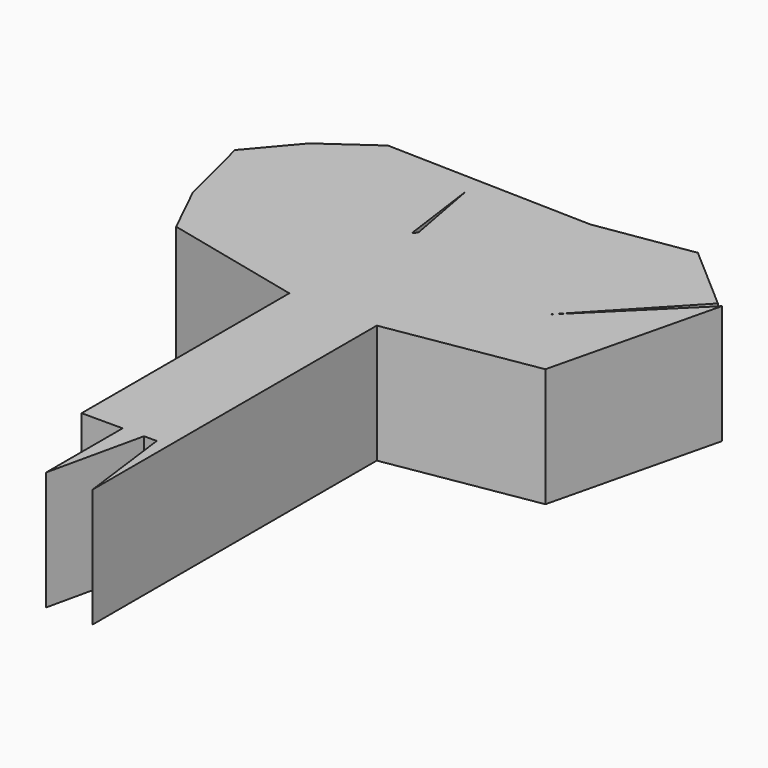
from build123d import *

# Parameters (mm, degrees)
F1_DEPTH = 25.4


with BuildPart() as f1:
    # F0 (on Top) → F1 (new body)
    with BuildSketch(Plane.XY):
        Polygon((-9.9282488227, 16.6444163769), (-9.9282488227, -38.8369709253), (-6.8141991987, -38.8369709253), (-4.3801111169, -38.8369709253), (-1.1680317111, -38.8369709253), (3.4067514008, -38.8369709253), (6.1321551912, -38.8369709253), (8.7602203712, -38.8369709253), (8.7602203712, 16.6444163769), (0, 16.6444163769), (-3.5040895455, 16.6444163769), (-6.8141991987, 16.6444163769), align=None)
        Polygon((-20.4405128956, 23.6525926739), (-9.9282488227, 16.6444163769), (-6.8141991987, 16.6444163769), (-12.2392783805, 23.6525926739), (-12.264306657, 23.6525926739), align=None)
        Polygon((-39.7129952908, 23.6525926739), (-9.9282488227, 16.6444163769), (-20.4405128956, 23.6525926739), align=None)
        Polygon((-12.2392783805, 23.6525926739), (-6.8141991987, 16.6444163769), (-3.5040895455, 16.6444163769), (-6.6358093424, 39.7052673339), (0, 27.0106745884), (0, 40.0465349111), (0, 51.3932853937), (-6.2433463768, 67.9810519437), (-16.1107429013, 68.2416611761), (-23.2746789764, 63.9495998621), (-15.1843791828, 53.4984625885), (-21.9592093912, 36.2089052796), (-18.098320559, 31.2213670903), align=None)
        Polygon((-6.8141991987, 47.2179802464), (-7.5501442092, 46.4380983203), (-9.9282488227, 63.9495998621), align=None, mode=Mode.SUBTRACT)
        Polygon((-30.4814127266, 30.3465261318), (-20.4405128956, 23.6525926739), (-12.264306657, 23.6525926739), (-12.2392783805, 23.6525926739), (-18.098320559, 31.2213670903), (-30.4814127266, 32.9626211831), align=None)
        Polygon((-39.7129952908, 23.6525926739), (-20.4405128956, 23.6525926739), (-30.4814127266, 30.3465261318), (-30.4814127266, 32.9626211831), (-45.2611297369, 35.0408777595), align=None)
        Polygon((3.4067514008, -38.8369709253), (-1.1680317111, -38.8369709253), (-1.1680317111, -59.2774823308), align=None)
        Polygon((-6.6358093424, 39.7052673339), (-3.5040895455, 16.6444163769), (0, 16.6444163769), (0, 21.9005476683), (0, 27.0106745884), align=None)
        Polygon((-49.3492335081, 51.3932853937), (-45.2611297369, 35.0408777595), (-30.4814127266, 32.9626211831), (-18.098320559, 31.2213670903), (-21.9592093912, 36.2089052796), (-30.4814127266, 47.2179802464), align=None)
        Polygon((0, 21.9005476683), (0, 16.6444163769), (8.7602203712, 16.6444163769), (15.9789933035, 43.8407290326), (18.5424652882, 53.4984625885), (21.3165320456, 63.9495998621), (34.1648571193, 70.665769279), (13.7243429199, 67.4536824226), (0, 56.9414235651), (0, 51.3932853937), (0, 40.0465349111), (0, 27.0106745884), align=None)
        Polygon((-41.173029691, 61.0295273364), (-49.3492335081, 51.3932853937), (-30.4814127266, 47.2179802464), (-33.7135461765, 51.3932853937), align=None)
        Polygon((8.7602203712, -38.8369709253), (6.1321551912, -38.8369709253), (8.7602203712, -59.2774823308), align=None)
        Polygon((15.9789933035, 43.8407290326), (8.7602203712, 16.6444163769), (18.5424652882, 27.0106745884), (28.3247102052, 37.3769327998), (38.2691381014, 47.9150565343), (48.2135659976, 58.4531802689), (34.1648571193, 70.665769279), (21.3165320456, 63.9495998621), (18.5424652882, 53.4984625885), align=None)
        Polygon((18.5424652882, 27.0106745884), (8.7602203712, 16.6444163769), (40.5890159309, 21.9005476683), (49.3492297828, 58.1094510853), (28.3247102052, 37.3769327998), align=None)
        Polygon((-30.4814127266, 47.2179802464), (-21.9592093912, 36.2089052796), (-15.1843791828, 53.4984625885), (-23.2746789764, 63.9495998621), (-16.1107429013, 68.2416611761), (-30.4322889094, 68.6199095927), (-33.7135461765, 51.3932853937), align=None)
        Polygon((-30.4322889094, 68.6199095927), (-41.173029691, 61.0295273364), (-33.7135461765, 51.3932853937), align=None)
        Polygon((-6.2433463768, 67.9810519437), (0, 51.3932853937), (0, 56.9414235651), (0, 67.8161580224), align=None)
        Polygon((0, 67.8161580224), (0, 56.9414235651), (13.7243429199, 67.4536824226), align=None)
    extrude(amount=F1_DEPTH)


solid = f1.part
